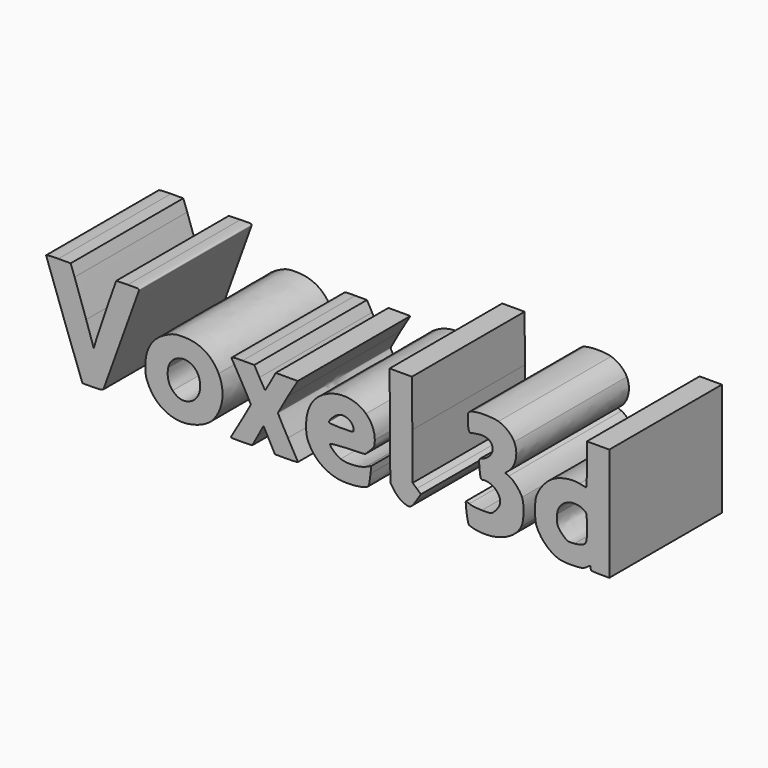
from build123d import *

# Parameters (mm, degrees)
F1_DEPTH = 25.4


# Not quite as in the source:
# - ends of sketch curves that miss each other by under 0.0002 mm in the source are joined


with BuildPart() as f1:
    # F0 (on Front) → F1 (new body)
    with BuildSketch(Plane.XZ):
        with BuildLine():
            add(Edge.make_bspline(
                [(-27.4528332055, -20.6560848736), (-29.6221518806, -20.2052889036), (-31.2485120431, -18.9675251212), (-32.2163183265, -17.0307712364)],
                knots=[0, 0, 0, 0, 1, 1, 1, 1], degree=3))
            add(Edge.make_bspline(
                [(-20.682280063, -18.5788280366), (-21.9881693371, -20.1227872817), (-25.231163843, -21.1177636457), (-27.4528332055, -20.6560848736)],
                knots=[0, 0, 0, 0, 1, 1, 1, 1], degree=3))
            add(Edge.make_bspline(
                [(-19.6846607646, -10.9128415954), (-18.4463352747, -13.4282347246), (-18.8319149947, -16.3911386184), (-20.682280063, -18.5788280366)],
                knots=[0, 0, 0, 0, 1, 1, 1, 1], degree=3))
            add(Edge.make_bspline(
                [(-25.9961221223, -7.1463693077), (-23.0609388272, -7.1463693077), (-20.905709834, -8.4325383981), (-19.6846607646, -10.9128415954)],
                knots=[0, 0, 0, 0, 1, 1, 1, 1], degree=3))
            add(Edge.make_bspline(
                [(-29.1742159191, -7.866766954), (-27.9120861176, -7.2454245155), (-27.4751000947, -7.1463693077), (-25.9961221223, -7.1463693077)],
                knots=[0, 0, 0, 0, 1, 1, 1, 1], degree=3))
            add(Edge.make_bspline(
                [(-32.8957538481, -13.9626557314), (-32.8875184559, -11.1139261514), (-31.6488751873, -9.0850388163), (-29.1742159191, -7.866766954)],
                knots=[0, 0, 0, 0, 1, 1, 1, 1], degree=3))
            add(Edge.make_bspline(
                [(-32.2163183265, -17.0307712364), (-32.8015257438, -15.8596671353), (-32.8999565836, -15.4151886958), (-32.8957538481, -13.9626557314)],
                knots=[0, 0, 0, 0, 1, 1, 1, 1], degree=3))
        make_face()
        with BuildLine():
            add(Edge.make_bspline(
                [(-24.7138133719, -16.9397634389), (-22.4077580939, -15.8454677973), (-22.430855236, -12.0284754067), (-24.7501923218, -10.9278778998)],
                knots=[0, 0, 0, 0, 1, 1, 1, 1], degree=3))
            add(Edge.make_bspline(
                [(-27.9619930419, -16.3080529102), (-26.9725106691, -17.3289394294), (-25.9521343861, -17.527383289), (-24.7138133719, -16.9397634389)],
                knots=[0, 0, 0, 0, 1, 1, 1, 1], degree=3))
            add(Edge.make_bspline(
                [(-28.7810251749, -12.9656115678), (-29.0361455407, -14.3255277002), (-28.7494240952, -15.4956314697), (-27.9619930419, -16.3080529102)],
                knots=[0, 0, 0, 0, 1, 1, 1, 1], degree=3))
            add(Edge.make_bspline(
                [(-24.7501923218, -10.9278778998), (-26.410102756, -10.1401984419), (-28.4438530007, -11.168333449), (-28.7810251749, -12.9656115678)],
                knots=[0, 0, 0, 0, 1, 1, 1, 1], degree=3))
        make_face(mode=Mode.SUBTRACT)
    extrude(amount=F1_DEPTH)


with BuildPart() as f1b:
    # F0 (on Front) → F1, piece 2 (new body)
    with BuildSketch(Plane.XZ):
        with BuildLine():
            add(Edge.make_bspline(
                [(1.9812820556, -20.6657099882), (-0.4464019088, -20.2237939194), (-2.3488267403, -18.8227299184), (-3.3729089497, -16.722548256)],
                knots=[0, 0, 0, 0, 1, 1, 1, 1], degree=3))
            add(Edge.make_bspline(
                [(6.5401937683, -20.4280517869), (5.3365039211, -20.7724523081), (3.184085703, -20.8846595268), (1.9812820556, -20.6657099882)],
                knots=[0, 0, 0, 0, 1, 1, 1, 1], degree=3))
            add(Edge.make_bspline(
                [(7.7204351266, -17.9204666151), (7.4847775885, -20.0915621656), (7.448758937, -20.1680931282), (6.5401937683, -20.4280517869)],
                knots=[0, 0, 0, 0, 1, 1, 1, 1], degree=3))
            Line((7.7204351266, -17.9204666151), (7.8594789821, -16.6394670236))
            Line((7.8594789821, -16.6394670236), (6.8420566985, -17.0895200179))
            add(Edge.make_bspline(
                [(2.3459152346, -17.3025257517), (3.4133294819, -17.7087789916), (5.6854630004, -17.6011370447), (6.8420566985, -17.0895200179)],
                knots=[0, 0, 0, 0, 1, 1, 1, 1], degree=3))
            add(Edge.make_bspline(
                [(0.4437186668, -15.610293641), (0.4437186668, -16.0008101206), (1.5787280285, -17.0105385785), (2.3459152346, -17.3025257517)],
                knots=[0, 0, 0, 0, 1, 1, 1, 1], degree=3))
            add(Edge.make_bspline(
                [(3.5925857728, -15.2345382067), (1.397220432, -15.3134905537), (0.4437186668, -15.4272710008), (0.4437186668, -15.610293641)],
                knots=[0, 0, 0, 0, 1, 1, 1, 1], degree=3))
            Line((3.5925857728, -15.2345382067), (6.7414528789, -15.1212970882))
            Line((6.7414528789, -15.1212970882), (7.6207667401, -14.2626701741))
            add(Edge.make_bspline(
                [(8.4951662205, -12.2745726471), (8.4996195984, -13.2969115493), (8.4166771144, -13.4854841277), (7.6207667401, -14.2626701741)],
                knots=[0, 0, 0, 0, 1, 1, 1, 1], degree=3))
            add(Edge.make_bspline(
                [(6.9049455549, -8.6388327348), (7.9179883106, -9.5999634273), (8.4892112263, -10.9059601196), (8.4951662205, -12.2745726471)],
                knots=[0, 0, 0, 0, 1, 1, 1, 1], degree=3))
            add(Edge.make_bspline(
                [(-0.3007742154, -7.8643992787), (2.2042955812, -6.6311560105), (5.119015717, -6.9444164549), (6.9049455549, -8.6388327348)],
                knots=[0, 0, 0, 0, 1, 1, 1, 1], degree=3))
            add(Edge.make_bspline(
                [(-3.8970312405, -13.942452166), (-3.8746748362, -11.0736331523), (-2.6642937327, -9.0279550163), (-0.3007742154, -7.8643992787)],
                knots=[0, 0, 0, 0, 1, 1, 1, 1], degree=3))
            add(Edge.make_bspline(
                [(-3.3729089497, -16.722548256), (-3.8000885898, -15.8464927456), (-3.9074306611, -15.2771138417), (-3.8970312405, -13.942452166)],
                knots=[0, 0, 0, 0, 1, 1, 1, 1], degree=3))
        make_face()
        with BuildLine():
            add(Edge.make_bspline(
                [(4.6956874656, -11.9781567128), (4.6956874656, -10.8262178016), (3.311203905, -9.9694169962), (2.0972153417, -10.3700688267)],
                knots=[0, 0, 0, 0, 1, 1, 1, 1], degree=3))
            add(Edge.make_bspline(
                [(2.4578091504, -12.3759373454), (4.4531171213, -12.3759373454), (4.6956874656, -12.3328201439), (4.6956874656, -11.9781567128)],
                knots=[0, 0, 0, 0, 1, 1, 1, 1], degree=3))
            add(Edge.make_bspline(
                [(0.2199308353, -12.1693207542), (0.2199308353, -12.282960215), (1.2269760771, -12.3759373454), (2.4578091504, -12.3759373454)],
                knots=[0, 0, 0, 0, 1, 1, 1, 1], degree=3))
            add(Edge.make_bspline(
                [(2.0972153417, -10.3700688267), (1.391408662, -10.6030051048), (0.2199308353, -11.7257889373), (0.2199308353, -12.1693207542)],
                knots=[0, 0, 0, 0, 1, 1, 1, 1], degree=3))
        make_face(mode=Mode.SUBTRACT)
    extrude(amount=F1_DEPTH)


with BuildPart() as f1c:
    # F0 (on Front) → F1, piece 3 (new body)
    with BuildSketch(Plane.XZ):
        with BuildLine():
            add(Edge.make_bspline(
                [(13.3669176566, -20.4167818317), (12.9050531405, -20.1729582756), (12.2504737333, -19.5555343621), (11.9122967517, -19.0447274473)],
                knots=[0, 0, 0, 0, 1, 1, 1, 1], degree=3))
            add(Edge.make_bspline(
                [(15.9579264562, -19.5471378427), (15.0048633151, -21.0264559726), (14.7095573684, -21.1255716032), (13.3669176566, -20.4167818317)],
                knots=[0, 0, 0, 0, 1, 1, 1, 1], degree=3))
            Line((15.9579264562, -19.5471378427), (16.8140312814, -18.2183125537))
            Line((16.8140312814, -18.2183125537), (16.069820372, -17.5535642274))
            Line((16.069820372, -17.5535642274), (15.3256094625, -16.8888159012))
            Line((15.3256094625, -16.8888159012), (15.2618791638, -8.4782112566))
            Line((15.2618791638, -8.4782112566), (15.1981466273, -0.0676066121))
            Line((15.1981466273, -0.0676066121), (13.1823038849, -0.0676066121))
            Line((13.1823038849, -0.0676066121), (11.1664611426, -0.0676066121))
            Line((11.1664611426, -0.0676066121), (11.2319437, -9.091794971))
            Line((11.2319437, -9.091794971), (11.2974284952, -18.1159855677))
            Line((11.2974284952, -18.1159855677), (11.9122967517, -19.0447274473))
        make_face()
    extrude(amount=F1_DEPTH)


with BuildPart() as f1d:
    # F0 (on Front) → F1, piece 4 (new body)
    with BuildSketch(Plane.XZ):
        with BuildLine():
            add(Edge.make_bspline(
                [(26.7641552204, -20.6531577287), (26.1626896172, -20.5472792299), (25.5757478442, -20.3658186288), (25.4598414126, -20.2499121973)],
                knots=[0, 0, 0, 0, 1, 1, 1, 1], degree=3))
            add(Edge.make_bspline(
                [(34.9325274404, -17.4235994443), (33.8407337468, -19.8273023047), (30.2154133959, -21.2606320353), (26.7641552204, -20.6531577287)],
                knots=[0, 0, 0, 0, 1, 1, 1, 1], degree=3))
            add(Edge.make_bspline(
                [(35.0469344935, -12.7440504252), (35.4939238324, -13.8138502508), (35.4325880636, -16.3226617799), (34.9325274404, -17.4235994443)],
                knots=[0, 0, 0, 0, 1, 1, 1, 1], degree=3))
            add(Edge.make_bspline(
                [(32.6803132768, -10.142624302), (33.4782802612, -10.4731522155), (34.6245551024, -11.7331560327), (35.0469344935, -12.7440504252)],
                knots=[0, 0, 0, 0, 1, 1, 1, 1], degree=3))
            Line((32.6803132768, -10.142624302), (32.0180355682, -9.8682984645))
            Line((32.0180355682, -9.8682984645), (32.6525501584, -9.3343899318))
            add(Edge.make_bspline(
                [(33.6470297135, -4.4015287527), (34.4097747311, -6.0088960419), (33.9613710531, -8.2330897312), (32.6525501584, -9.3343899318)],
                knots=[0, 0, 0, 0, 1, 1, 1, 1], degree=3))
            add(Edge.make_bspline(
                [(30.8103264915, -2.087173184), (31.9931794537, -2.4420380242), (33.1745666057, -3.4058855009), (33.6470297135, -4.4015287527)],
                knots=[0, 0, 0, 0, 1, 1, 1, 1], degree=3))
            add(Edge.make_bspline(
                [(26.0515095846, -2.0869493961), (27.0936872781, -1.7430009264), (29.663431758, -1.7431486263), (30.8103264915, -2.087173184)],
                knots=[0, 0, 0, 0, 1, 1, 1, 1], degree=3))
            add(Edge.make_bspline(
                [(25.2872226688, -3.497725789), (25.2842686694, -2.3768754834), (25.3084825128, -2.3321716262), (26.0515095846, -2.0869493961)],
                knots=[0, 0, 0, 0, 1, 1, 1, 1], degree=3))
            add(Edge.make_bspline(
                [(25.9289946984, -5.5338526604), (25.4804701749, -5.7242535854), (25.2915193952, -5.1247774559), (25.2872226688, -3.497725789)],
                knots=[0, 0, 0, 0, 1, 1, 1, 1], degree=3))
            add(Edge.make_bspline(
                [(27.4101523643, -5.2754090453), (26.7947358276, -5.3329829407), (26.1282151018, -5.449281001), (25.9289946984, -5.5338526604)],
                knots=[0, 0, 0, 0, 1, 1, 1, 1], degree=3))
            add(Edge.make_bspline(
                [(29.7599245952, -6.8894854938), (29.7599245952, -5.7533213868), (28.8659190628, -5.1392229605), (27.4101523643, -5.2754090453)],
                knots=[0, 0, 0, 0, 1, 1, 1, 1], degree=3))
            add(Edge.make_bspline(
                [(27.8404806991, -8.9315516942), (28.8497750087, -8.6782350583), (29.7599245952, -7.7099409174), (29.7599245952, -6.8894854938)],
                knots=[0, 0, 0, 0, 1, 1, 1, 1], degree=3))
            add(Edge.make_bspline(
                [(27.4453318114, -11.2184619232), (27.2120240455, -9.2756769564), (27.245688449, -9.080833843), (27.8404806991, -8.9315516942)],
                knots=[0, 0, 0, 0, 1, 1, 1, 1], degree=3))
            add(Edge.make_bspline(
                [(28.0082723395, -12.3009885628), (27.6482223352, -12.3951428171), (27.5681465733, -12.241158886), (27.4453318114, -11.2184619232)],
                knots=[0, 0, 0, 0, 1, 1, 1, 1], degree=3))
            add(Edge.make_bspline(
                [(30.5287969237, -13.2948057059), (29.931457968, -12.5849081846), (28.731626223, -12.1118274224), (28.0082723395, -12.3009885628)],
                knots=[0, 0, 0, 0, 1, 1, 1, 1], degree=3))
            add(Edge.make_bspline(
                [(30.3363662431, -16.3514565602), (31.3014893105, -15.2986355174), (31.3650719091, -14.2886608929), (30.5287969237, -13.2948057059)],
                knots=[0, 0, 0, 0, 1, 1, 1, 1], degree=3))
            add(Edge.make_bspline(
                [(27.8187531386, -17.1763138905), (29.56073776, -17.1873242518), (29.5741695056, -17.1829156315), (30.3363662431, -16.3514565602)],
                knots=[0, 0, 0, 0, 1, 1, 1, 1], degree=3))
            add(Edge.make_bspline(
                [(25.5447353265, -16.878447811), (25.8377161177, -17.0392102755), (26.8370876747, -17.1701127297), (27.8187531386, -17.1763138905)],
                knots=[0, 0, 0, 0, 1, 1, 1, 1], degree=3))
            add(Edge.make_bspline(
                [(24.9306100456, -16.6830787962), (24.9808996471, -16.6327891947), (25.2572574782, -16.7207042443), (25.5447353265, -16.878447811)],
                knots=[0, 0, 0, 0, 1, 1, 1, 1], degree=3))
            add(Edge.make_bspline(
                [(25.4598414126, -20.2499121973), (25.2416326118, -20.0317033964), (24.7687890647, -16.8448997771), (24.9306100456, -16.6830787962)],
                knots=[0, 0, 0, 0, 1, 1, 1, 1], degree=3))
        make_face()
    extrude(amount=F1_DEPTH)


with BuildPart() as f1e:
    # F0 (on Front) → F1, piece 5 (new body)
    with BuildSketch(Plane.XZ):
        with BuildLine():
            add(Edge.make_bspline(
                [(41.5642784183, -20.3476895766), (39.9341116248, -19.7447939691), (38.4170986725, -18.2562759214), (37.7113166095, -16.5671007525)],
                knots=[0, 0, 0, 0, 1, 1, 1, 1], degree=3))
            add(Edge.make_bspline(
                [(44.2316190094, -20.6012098594), (43.088824069, -20.6368614988), (42.0892913847, -20.5418590886), (41.5642784183, -20.3476895766)],
                knots=[0, 0, 0, 0, 1, 1, 1, 1], degree=3))
            add(Edge.make_bspline(
                [(46.7492321139, -20.0339703671), (46.1848257756, -20.4513637653), (45.7267701284, -20.5545657617), (44.2316190094, -20.6012098594)],
                knots=[0, 0, 0, 0, 1, 1, 1, 1], degree=3))
            add(Edge.make_bspline(
                [(47.4391632848, -19.9780234092), (47.4391632848, -19.533614344), (47.4241695001, -19.5348295119), (46.7492321139, -20.0339703671)],
                knots=[0, 0, 0, 0, 1, 1, 1, 1], degree=3))
            add(Edge.make_bspline(
                [(49.1175720212, -20.4322992799), (47.5801048611, -20.4322992799), (47.4391632848, -20.3941524062), (47.4391632848, -19.9780234092)],
                knots=[0, 0, 0, 0, 1, 1, 1, 1], degree=3))
            Line((49.1175720212, -20.4322992799), (50.7959807576, -20.4322992799))
            Line((50.7959807576, -20.4322992799), (50.7959807576, -10.249952946))
            Line((50.7959807576, -10.249952946), (50.7959807576, -0.0676066121))
            Line((50.7959807576, -0.0676066121), (48.7818902739, -0.0676066121))
            Line((48.7818902739, -0.0676066121), (46.7677997903, -0.0676066121))
            Line((46.7677997903, -0.0676066121), (46.7677997903, -3.7601058321))
            add(Edge.make_bspline(
                [(46.5999589167, -7.4471334396), (46.6922713972, -7.4501321965), (46.7677997903, -5.7909804031), (46.7677997903, -3.7601058321)],
                knots=[0, 0, 0, 0, 1, 1, 1, 1], degree=3))
            add(Edge.make_bspline(
                [(45.4324824163, -7.2113147743), (45.9822821229, -7.3380055414), (46.5076464362, -7.4441257312), (46.5999589167, -7.4471334396)],
                knots=[0, 0, 0, 0, 1, 1, 1, 1], degree=3))
            add(Edge.make_bspline(
                [(40.3641960309, -8.1970352736), (41.7328443645, -7.3029402261), (43.9547755588, -6.8707992098), (45.4324824163, -7.2113147743)],
                knots=[0, 0, 0, 0, 1, 1, 1, 1], degree=3))
            add(Edge.make_bspline(
                [(37.5997740406, -11.888681862), (37.9591907253, -10.594633202), (39.1707825209, -8.9766561317), (40.3641960309, -8.1970352736)],
                knots=[0, 0, 0, 0, 1, 1, 1, 1], degree=3))
            add(Edge.make_bspline(
                [(37.7113166095, -16.5671007525), (37.3188688409, -15.627838607), (37.2589742656, -13.1157060664), (37.5997740406, -11.888681862)],
                knots=[0, 0, 0, 0, 1, 1, 1, 1], degree=3))
        make_face()
        with BuildLine():
            add(Edge.make_bspline(
                [(46.3118387972, -16.5236008738), (46.7144935288, -16.159202672), (46.7677997903, -15.840913715), (46.7677997903, -13.8010339216)],
                knots=[0, 0, 0, 0, 1, 1, 1, 1], degree=3))
            add(Edge.make_bspline(
                [(44.5220665223, -17.0327204284), (45.3970993223, -16.969426516), (46.0127083165, -16.7943102999), (46.3118387972, -16.5236008738)],
                knots=[0, 0, 0, 0, 1, 1, 1, 1], degree=3))
            add(Edge.make_bspline(
                [(42.2925735372, -16.2335181351), (43.1708960183, -17.1118406162), (43.2141072107, -17.127328972), (44.5220665223, -17.0327204284)],
                knots=[0, 0, 0, 0, 1, 1, 1, 1], degree=3))
            add(Edge.make_bspline(
                [(41.3844716093, -13.3865743819), (41.259161613, -14.9059482958), (41.3969365915, -15.3378811894), (42.2925735372, -16.2335181351)],
                knots=[0, 0, 0, 0, 1, 1, 1, 1], degree=3))
            add(Edge.make_bspline(
                [(46.2642771694, -11.1753805278), (44.2545796409, -9.9152446758), (41.5704572003, -11.1315046856), (41.3844716093, -13.3865743819)],
                knots=[0, 0, 0, 0, 1, 1, 1, 1], degree=3))
            add(Edge.make_bspline(
                [(46.7677997903, -13.8010339216), (46.7677997903, -11.6482912112), (46.7335356354, -11.4696190066), (46.2642771694, -11.1753805278)],
                knots=[0, 0, 0, 0, 1, 1, 1, 1], degree=3))
        make_face(mode=Mode.SUBTRACT)
    extrude(amount=F1_DEPTH)


with BuildPart() as f1f:
    # F0 (on Front) → F1, piece 6 (new body)
    with BuildSketch(Plane.XZ):
        with BuildLine():
            add(Edge.make_bspline(
                [(-47.5284300389, -11.4248390615), (-49.3301839144, -6.4707359413), (-50.8041982727, -2.3418504499), (-50.8040192424, -2.2495379694)],
                knots=[0, 0, 0, 0, 1, 1, 1, 1], degree=3))
            Line((-47.5284300389, -11.4248390615), (-44.252516343, -20.4322992799))
            Line((-44.252516343, -20.4322992799), (-42.4049284818, -20.4322992799))
            add(Edge.make_bspline(
                [(-40.4505826356, -20.1525644905), (-40.5240790352, -20.3451428711), (-41.1329878217, -20.4322992799), (-42.4049284818, -20.4322992799)],
                knots=[0, 0, 0, 0, 1, 1, 1, 1], degree=3))
            add(Edge.make_bspline(
                [(-34.0711211074, -2.4645533179), (-34.1543589913, -2.772283965), (-39.9455740635, -18.8293003292), (-40.4505826356, -20.1525644905)],
                knots=[0, 0, 0, 0, 1, 1, 1, 1], degree=3))
            add(Edge.make_bspline(
                [(-36.060514366, -2.1288715706), (-34.1372101298, -2.0695297513), (-33.9718219708, -2.0974383318), (-34.0711211074, -2.4645533179)],
                knots=[0, 0, 0, 0, 1, 1, 1, 1], degree=3))
            Line((-36.060514366, -2.1288715706), (-38.1582097456, -2.1935910115))
            Line((-38.1582097456, -2.1935910115), (-39.6560642216, -6.4455598103))
            add(Edge.make_bspline(
                [(-41.6781842126, -12.4553976907), (-41.3898380675, -11.4885693601), (-40.4798854142, -8.7841426496), (-39.6560642216, -6.4455598103)],
                knots=[0, 0, 0, 0, 1, 1, 1, 1], degree=3))
            Line((-41.6781842126, -12.4553976907), (-42.2024497276, -14.2132690103))
            Line((-42.2024497276, -14.2132690103), (-43.5730405396, -10.1056254598))
            add(Edge.make_bspline(
                [(-45.6569483509, -4.0398406215), (-45.2646236656, -5.1168195607), (-44.3268653743, -7.8464224022), (-43.5730405396, -10.1056254598)],
                knots=[0, 0, 0, 0, 1, 1, 1, 1], degree=3))
            Line((-45.6569483509, -4.0398406215), (-46.3702675881, -2.0816970957))
            Line((-46.3702675881, -2.0816970957), (-48.5869800502, -2.0816970957))
            add(Edge.make_bspline(
                [(-50.8040192424, -2.2495379694), (-50.8038402122, -2.1572254889), (-49.8061739184, -2.0816970957), (-48.5869800502, -2.0816970957)],
                knots=[0, 0, 0, 0, 1, 1, 1, 1], degree=3))
        make_face()
    extrude(amount=F1_DEPTH)


with BuildPart() as f1g:
    # F0 (on Front) → F1, piece 7 (new body)
    with BuildSketch(Plane.XZ):
        with BuildLine():
            add(Edge.make_bspline(
                [(-17.4593078544, -20.3152179622), (-17.4593078544, -20.2412381809), (-16.6536716609, -18.8275771629), (-15.6690052023, -17.173747044)],
                knots=[0, 0, 0, 0, 1, 1, 1, 1], degree=3))
            add(Edge.make_bspline(
                [(-15.5275041564, -20.3850643823), (-16.5899950714, -20.4206287445), (-17.4593078544, -20.3892044572), (-17.4593078544, -20.3152179622)],
                knots=[0, 0, 0, 0, 1, 1, 1, 1], degree=3))
            Line((-15.5275041564, -20.3850643823), (-13.5956982206, -20.3204053642))
            Line((-13.5956982206, -20.3204053642), (-12.5873997669, -18.4548025825))
            Line((-12.5873997669, -18.4548025825), (-11.5790990753, -16.589197563))
            Line((-11.5790990753, -16.589197563), (-10.5486590536, -18.5107495404))
            Line((-10.5486590536, -18.5107495404), (-9.5182190319, -20.4322992799))
            Line((-9.5182190319, -20.4322992799), (-7.4464919922, -20.4322992799))
            add(Edge.make_bspline(
                [(-5.3747649526, -20.31135986), (-5.3747649526, -20.3778763172), (-6.3070426799, -20.4322992799), (-7.4464919922, -20.4322992799)],
                knots=[0, 0, 0, 0, 1, 1, 1, 1], degree=3))
            add(Edge.make_bspline(
                [(-7.1650676047, -17.0754818072), (-6.1804011461, -18.7886985029), (-5.3747649526, -20.2448434029), (-5.3747649526, -20.31135986)],
                knots=[0, 0, 0, 0, 1, 1, 1, 1], degree=3))
            add(Edge.make_bspline(
                [(-8.9553702568, -13.6974179178), (-8.9553702568, -13.8421370327), (-8.1497340634, -15.3622651115), (-7.1650676047, -17.0754818072)],
                knots=[0, 0, 0, 0, 1, 1, 1, 1], degree=3))
            add(Edge.make_bspline(
                [(-7.1795063956, -10.4434488567), (-8.1562306241, -12.0884125016), (-8.9553702568, -13.5526988029), (-8.9553702568, -13.6974179178)],
                knots=[0, 0, 0, 0, 1, 1, 1, 1], degree=3))
            Line((-7.1795063956, -10.4434488567), (-5.4036402965, -7.4526050521))
            Line((-5.4036402965, -7.4526050521), (-7.3876178895, -7.4526050521))
            Line((-7.3876178895, -7.4526050521), (-9.3715954826, -7.4526050521))
            Line((-9.3715954826, -7.4526050521), (-10.2980972459, -9.1310137884))
            add(Edge.make_bspline(
                [(-11.3051424877, -10.8094225248), (-11.2608436865, -10.8094225248), (-10.8076733277, -10.0541385934), (-10.2980972459, -9.1310137884)],
                knots=[0, 0, 0, 0, 1, 1, 1, 1], degree=3))
            add(Edge.make_bspline(
                [(-12.3121877296, -9.1310137884), (-11.8026116478, -10.0541385934), (-11.349441289, -10.8094225248), (-11.3051424877, -10.8094225248)],
                knots=[0, 0, 0, 0, 1, 1, 1, 1], degree=3))
            Line((-12.3121877296, -9.1310137884), (-13.2386894929, -7.4526050521))
            Line((-13.2386894929, -7.4526050521), (-15.3568726485, -7.4526050521))
            add(Edge.make_bspline(
                [(-17.2645430668, -7.8442337572), (-17.4581732501, -7.4840114364), (-17.3051918885, -7.4526050521), (-15.3568726485, -7.4526050521)],
                knots=[0, 0, 0, 0, 1, 1, 1, 1], degree=3))
            add(Edge.make_bspline(
                [(-15.4663675587, -10.9980443365), (-16.3395832015, -9.4788449771), (-17.1487619564, -8.0596295451), (-17.2645430668, -7.8442337572)],
                knots=[0, 0, 0, 0, 1, 1, 1, 1], degree=3))
            add(Edge.make_bspline(
                [(-13.8787025502, -13.9635038873), (-13.8787025502, -13.8517017246), (-14.5931519159, -12.5172459337), (-15.4663675587, -10.9980443365)],
                knots=[0, 0, 0, 0, 1, 1, 1, 1], degree=3))
            add(Edge.make_bspline(
                [(-15.6690052023, -17.173747044), (-14.6843387436, -15.5199169252), (-13.8787025502, -14.0753082879), (-13.8787025502, -13.9635038873)],
                knots=[0, 0, 0, 0, 1, 1, 1, 1], degree=3))
        make_face()
    extrude(amount=F1_DEPTH)


solid = Compound([f1.part, f1b.part, f1c.part, f1d.part, f1e.part, f1f.part, f1g.part])
